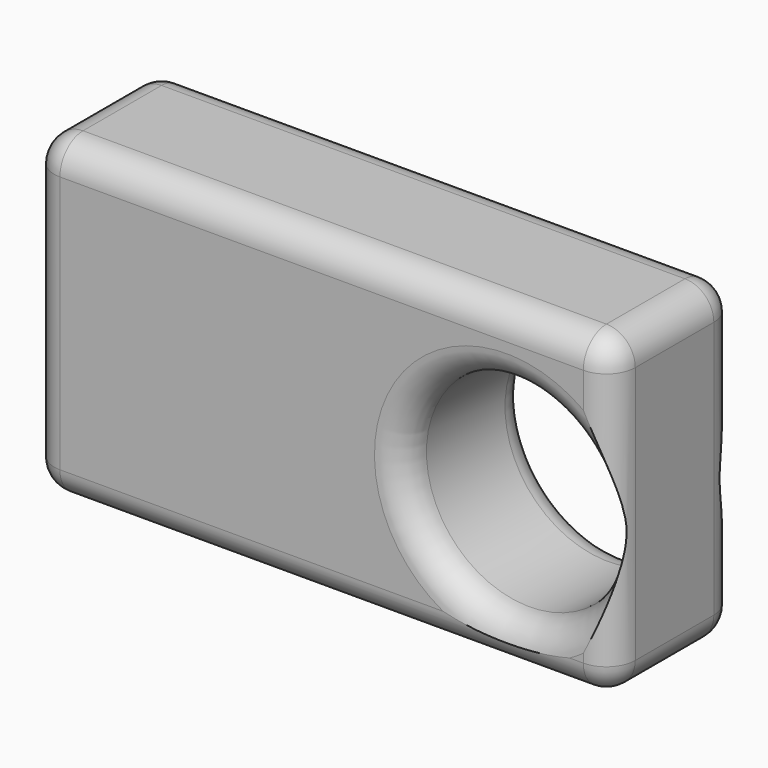
from build123d import *

# Parameters (mm, degrees)
F0_W         = 102.2414937615
F0_H         = 55.510988459
F0_R         = 18.1160237287
F1_DEPTH     = 27.432
F2_T1_DEPTH  = 92.0814937615
F2_T3_DEPTH  = 45.350988459
F2_T5_DEPTH  = 17.272
F2_S9_W      = 5.08
F2_S9_H      = 5.08
F2_T10_DEPTH = 5.08
F2_S15_W     = 5.08
F2_S15_H     = 5.08
F2_T16_DEPTH = 5.08
F2_S21_W     = 5.08
F2_S21_H     = 5.08
F2_T22_DEPTH = 5.08
F2_S27_W     = 5.08
F2_S27_H     = 5.08
F2_T28_DEPTH = 5.08
F2_S33_W     = 5.08
F2_S33_H     = 5.08
F2_T34_DEPTH = 5.08
F2_S39_W     = 5.08
F2_S39_H     = 5.08
F2_T40_DEPTH = 5.08
F2_S45_W     = 5.08
F2_S45_H     = 5.08
F2_T46_DEPTH = 5.08
F2_S51_W     = 5.08
F2_S51_H     = 5.08
F2_T52_DEPTH = 5.08


# Not quite as in the source:
# - a fillet or chamfer that OpenCascade refuses, or shapes differently, is made with other operations: its cross-section is extruded or revolved along the edge and cut away or added


with BuildPart() as f1:
    # F0 (on Front) → F1 (new body)
    with BuildSketch(Plane.XZ):
        with Locations((-13.5455615819, 6.0090096667)):
            Rectangle(F0_W, F0_H)
        with Locations((18.9486481249, 3.6901270505)):
            Circle(F0_R, mode=Mode.SUBTRACT)
    extrude(amount=F1_DEPTH)

    # F2: fillet of radius 5.08 on 15 edges, made by hand

    # F2_s2 → F2_t1 (cut)
    with BuildSketch(Plane.YZ.offset(-59.5863084626)):
        with BuildLine():
            ThreePointArc((-22.352, 33.7645038962), (-25.9441024484, 32.2766063447), (-27.432, 28.6845038962))
            Line((-27.432, 28.6845038962), (-27.432, 33.7645038962))
            Line((-27.432, 33.7645038962), (-22.352, 33.7645038962))
        make_face()
        with BuildLine():
            ThreePointArc((-22.352, -21.7464845628), (-25.9441024484, -20.2585870112), (-27.432, -16.6664845628))
            Line((-27.432, -16.6664845628), (-27.432, -21.7464845628))
            Line((-27.432, -21.7464845628), (-22.352, -21.7464845628))
        make_face()
        with BuildLine():
            ThreePointArc((-5.08, -21.7464845628), (-1.4878975516, -20.2585870112), (0, -16.6664845628))
            Line((0, -16.6664845628), (0, -21.7464845628))
            Line((0, -21.7464845628), (-5.08, -21.7464845628))
        make_face()
        with BuildLine():
            ThreePointArc((-5.08, 33.7645038962), (-1.4878975516, 32.2766063447), (0, 28.6845038962))
            Line((0, 28.6845038962), (0, 33.7645038962))
            Line((0, 33.7645038962), (-5.08, 33.7645038962))
        make_face()
    extrude(amount=F2_T1_DEPTH, mode=Mode.SUBTRACT)

    # F2_s4 → F2_t3 (cut)
    with BuildSketch(Plane.XY.offset(-16.6664845628)):
        with BuildLine():
            ThreePointArc((-64.6663084626, -22.352), (-63.178410911, -25.9441024484), (-59.5863084626, -27.432))
            Line((-59.5863084626, -27.432), (-64.6663084626, -27.432))
            Line((-64.6663084626, -27.432), (-64.6663084626, -22.352))
        make_face()
        with BuildLine():
            ThreePointArc((37.5751852989, -22.352), (36.0872877473, -25.9441024484), (32.4951852989, -27.432))
            Line((32.4951852989, -27.432), (37.5751852989, -27.432))
            Line((37.5751852989, -27.432), (37.5751852989, -22.352))
        make_face()
        with BuildLine():
            ThreePointArc((-64.6663084626, -5.08), (-63.178410911, -1.4878975516), (-59.5863084626, 0))
            Line((-59.5863084626, 0), (-64.6663084626, 0))
            Line((-64.6663084626, 0), (-64.6663084626, -5.08))
        make_face()
        with BuildLine():
            ThreePointArc((37.5751852989, -5.08), (36.0872877473, -1.4878975516), (32.4951852989, 0))
            Line((32.4951852989, 0), (37.5751852989, 0))
            Line((37.5751852989, 0), (37.5751852989, -5.08))
        make_face()
    extrude(amount=F2_T3_DEPTH, mode=Mode.SUBTRACT)

    # F2_s6 → F2_t5 (cut)
    with BuildSketch(Plane.XZ.offset(5.08)):
        with BuildLine():
            ThreePointArc((-64.6663084626, -16.6664845628), (-63.178410911, -20.2585870112), (-59.5863084626, -21.7464845628))
            Line((-59.5863084626, -21.7464845628), (-64.6663084626, -21.7464845628))
            Line((-64.6663084626, -21.7464845628), (-64.6663084626, -16.6664845628))
        make_face()
        with BuildLine():
            ThreePointArc((32.4951852989, -21.7464845628), (36.0872877473, -20.2585870112), (37.5751852989, -16.6664845628))
            Line((37.5751852989, -16.6664845628), (37.5751852989, -21.7464845628))
            Line((37.5751852989, -21.7464845628), (32.4951852989, -21.7464845628))
        make_face()
        with BuildLine():
            ThreePointArc((-59.5863084626, 33.7645038962), (-63.178410911, 32.2766063447), (-64.6663084626, 28.6845038962))
            Line((-64.6663084626, 28.6845038962), (-64.6663084626, 33.7645038962))
            Line((-64.6663084626, 33.7645038962), (-59.5863084626, 33.7645038962))
        make_face()
        with BuildLine():
            ThreePointArc((32.4951852989, 33.7645038962), (36.0872877473, 32.2766063447), (37.5751852989, 28.6845038962))
            Line((37.5751852989, 28.6845038962), (37.5751852989, 33.7645038962))
            Line((37.5751852989, 33.7645038962), (32.4951852989, 33.7645038962))
        make_face()
    extrude(amount=F2_T5_DEPTH, mode=Mode.SUBTRACT)


with BuildPart() as f2_tool8:
    # F2_s9 → F2_t10 (new body)
    with BuildSketch(Plane.XY.offset(28.6845038962)):
        with Locations((35.0351852989, -24.892)):
            Rectangle(F2_S9_W, F2_S9_H)
    extrude(amount=F2_T10_DEPTH)

    # F2_s11 → F2_t12 (revolve, cut)
    with BuildSketch(Plane(origin=(32.4951852989, -22.352, 28.6845038962), x_dir=(-0.7071067812, 0.7071067812, 0), z_dir=(0.7071067812, 0.7071067812, 0))):
        with BuildLine():
            ThreePointArc((0, -5.08), (5.08, 0), (0, 5.08))
            Line((0, 5.08), (0, -5.08))
        make_face()
    revolve(axis=Axis((32.4951852989, -22.352, 28.6845038962), (0, 0, 1)), mode=Mode.SUBTRACT)


with BuildPart() as f1_1:
    add(f1.part)

    # F2_t7: cut F2_tool8
    add(f2_tool8.part, mode=Mode.SUBTRACT)


with BuildPart() as f2_tool14:
    # F2_s15 → F2_t16 (new body)
    with BuildSketch(Plane.XY.offset(28.6845038962)):
        with Locations((-62.1263084626, -24.892)):
            Rectangle(F2_S15_W, F2_S15_H)
    extrude(amount=F2_T16_DEPTH)

    # F2_s17 → F2_t18 (revolve, cut)
    with BuildSketch(Plane(origin=(-59.5863084626, -22.352, 28.6845038962), x_dir=(0.7071067812, 0.7071067812, 0), z_dir=(0.7071067812, -0.7071067812, 0))):
        with BuildLine():
            ThreePointArc((0, -5.08), (5.08, 0), (0, 5.08))
            Line((0, 5.08), (0, -5.08))
        make_face()
    revolve(axis=Axis((-59.5863084626, -22.352, 28.6845038962), (0, 0, 1)), mode=Mode.SUBTRACT)


with BuildPart() as f1_2:
    add(f1_1.part)

    # F2_t13: cut F2_tool14
    add(f2_tool14.part, mode=Mode.SUBTRACT)


with BuildPart() as f2_tool20:
    # F2_s21 → F2_t22 (new body)
    with BuildSketch(Plane.YZ.offset(-59.5863084626)):
        with Locations((-24.892, -19.2064845628)):
            Rectangle(F2_S21_W, F2_S21_H)
    extrude(amount=-F2_T22_DEPTH)

    # F2_s23 → F2_t24 (revolve, cut)
    with BuildSketch(Plane(origin=(-59.5863084626, -22.352, -16.6664845628), x_dir=(0, 0.7071067812, 0.7071067812), z_dir=(0, -0.7071067812, 0.7071067812))):
        with BuildLine():
            ThreePointArc((0, -5.08), (5.08, 0), (0, 5.08))
            Line((0, 5.08), (0, -5.08))
        make_face()
    revolve(axis=Axis((-59.5863084626, -22.352, -16.6664845628), (-1, 0, 0)), mode=Mode.SUBTRACT)


with BuildPart() as f1_3:
    add(f1_2.part)

    # F2_t19: cut F2_tool20
    add(f2_tool20.part, mode=Mode.SUBTRACT)


with BuildPart() as f2_tool26:
    # F2_s27 → F2_t28 (new body)
    with BuildSketch(Plane.XY.offset(-16.6664845628)):
        with Locations((35.0351852989, -24.892)):
            Rectangle(F2_S27_W, F2_S27_H)
    extrude(amount=-F2_T28_DEPTH)

    # F2_s29 → F2_t30 (revolve, cut)
    with BuildSketch(Plane(origin=(32.4951852989, -22.352, -16.6664845628), x_dir=(-0.7071067812, 0.7071067812, 0), z_dir=(-0.7071067812, -0.7071067812, 0))):
        with BuildLine():
            ThreePointArc((0, -5.08), (5.08, 0), (0, 5.08))
            Line((0, 5.08), (0, -5.08))
        make_face()
    revolve(axis=Axis((32.4951852989, -22.352, -16.6664845628), (0, 0, -1)), mode=Mode.SUBTRACT)


with BuildPart() as f1_4:
    add(f1_3.part)

    # F2_t25: cut F2_tool26
    add(f2_tool26.part, mode=Mode.SUBTRACT)


with BuildPart() as f2_tool32:
    # F2_s33 → F2_t34 (new body)
    with BuildSketch(Plane.YZ.offset(-59.5863084626)):
        with Locations((-2.54, -19.2064845628)):
            Rectangle(F2_S33_W, F2_S33_H)
    extrude(amount=-F2_T34_DEPTH)

    # F2_s35 → F2_t36 (revolve, cut)
    with BuildSketch(Plane(origin=(-59.5863084626, -5.08, -16.6664845628), x_dir=(0, -0.7071067812, 0.7071067812), z_dir=(0, -0.7071067812, -0.7071067812))):
        with BuildLine():
            ThreePointArc((0, -5.08), (5.08, 0), (0, 5.08))
            Line((0, 5.08), (0, -5.08))
        make_face()
    revolve(axis=Axis((-59.5863084626, -5.08, -16.6664845628), (-1, 0, 0)), mode=Mode.SUBTRACT)


with BuildPart() as f1_5:
    add(f1_4.part)

    # F2_t31: cut F2_tool32
    add(f2_tool32.part, mode=Mode.SUBTRACT)


with BuildPart() as f2_tool38:
    # F2_s39 → F2_t40 (new body)
    with BuildSketch(Plane.XY.offset(-16.6664845628)):
        with Locations((35.0351852989, -2.54)):
            Rectangle(F2_S39_W, F2_S39_H)
    extrude(amount=-F2_T40_DEPTH)

    # F2_s41 → F2_t42 (revolve, cut)
    with BuildSketch(Plane(origin=(32.4951852989, -5.08, -16.6664845628), x_dir=(-0.7071067812, -0.7071067812, 0), z_dir=(0.7071067812, -0.7071067812, 0))):
        with BuildLine():
            ThreePointArc((0, -5.08), (5.08, 0), (0, 5.08))
            Line((0, 5.08), (0, -5.08))
        make_face()
    revolve(axis=Axis((32.4951852989, -5.08, -16.6664845628), (0, 0, -1)), mode=Mode.SUBTRACT)


with BuildPart() as f1_6:
    add(f1_5.part)

    # F2_t37: cut F2_tool38
    add(f2_tool38.part, mode=Mode.SUBTRACT)


with BuildPart() as f2_tool44:
    # F2_s45 → F2_t46 (new body)
    with BuildSketch(Plane.XY.offset(28.6845038962)):
        with Locations((35.0351852989, -2.54)):
            Rectangle(F2_S45_W, F2_S45_H)
    extrude(amount=F2_T46_DEPTH)

    # F2_s47 → F2_t48 (revolve, cut)
    with BuildSketch(Plane(origin=(32.4951852989, -5.08, 28.6845038962), x_dir=(-0.7071067812, -0.7071067812, 0), z_dir=(-0.7071067812, 0.7071067812, 0))):
        with BuildLine():
            ThreePointArc((0, -5.08), (5.08, 0), (0, 5.08))
            Line((0, 5.08), (0, -5.08))
        make_face()
    revolve(axis=Axis((32.4951852989, -5.08, 28.6845038962), (0, 0, 1)), mode=Mode.SUBTRACT)


with BuildPart() as f1_7:
    add(f1_6.part)

    # F2_t43: cut F2_tool44
    add(f2_tool44.part, mode=Mode.SUBTRACT)


with BuildPart() as f2_tool50:
    # F2_s51 → F2_t52 (new body)
    with BuildSketch(Plane.XY.offset(28.6845038962)):
        with Locations((-62.1263084626, -2.54)):
            Rectangle(F2_S51_W, F2_S51_H)
    extrude(amount=F2_T52_DEPTH)

    # F2_s53 → F2_t54 (revolve, cut)
    with BuildSketch(Plane(origin=(-59.5863084626, -5.08, 28.6845038962), x_dir=(0.7071067812, -0.7071067812, 0), z_dir=(-0.7071067812, -0.7071067812, 0))):
        with BuildLine():
            ThreePointArc((0, -5.08), (5.08, 0), (0, 5.08))
            Line((0, 5.08), (0, -5.08))
        make_face()
    revolve(axis=Axis((-59.5863084626, -5.08, 28.6845038962), (0, 0, 1)), mode=Mode.SUBTRACT)


with BuildPart() as f1_8:
    add(f1_7.part)

    # F2_t49: cut F2_tool50
    add(f2_tool50.part, mode=Mode.SUBTRACT)

    # F2_s55 → F2_t56 (revolve, cut)
    with BuildSketch(Plane.XY.offset(3.6901270505)):
        with BuildLine():
            ThreePointArc((37.0646718537, -22.352), (38.5525694052, -25.9441024484), (42.1446718537, -27.432))
            Line((42.1446718537, -27.432), (37.0646718537, -27.432))
            Line((37.0646718537, -27.432), (37.0646718537, -22.352))
        make_face()
    revolve(axis=Axis((18.9486481249, -27.432, 3.6901270505), (0, -1, 0)), mode=Mode.SUBTRACT)

    # F2_s57 → F2_t58 (revolve, cut)
    with BuildSketch(Plane.XY.offset(3.6901270505)):
        with BuildLine():
            ThreePointArc((37.0646718537, -5.08), (38.5525694052, -1.4878975516), (42.1446718537, 0))
            Line((42.1446718537, 0), (37.0646718537, 0))
            Line((37.0646718537, 0), (37.0646718537, -5.08))
        make_face()
    revolve(axis=Axis((18.9486481249, 0, 3.6901270505), (0, -1, 0)), mode=Mode.SUBTRACT)


solid = f1_8.part
